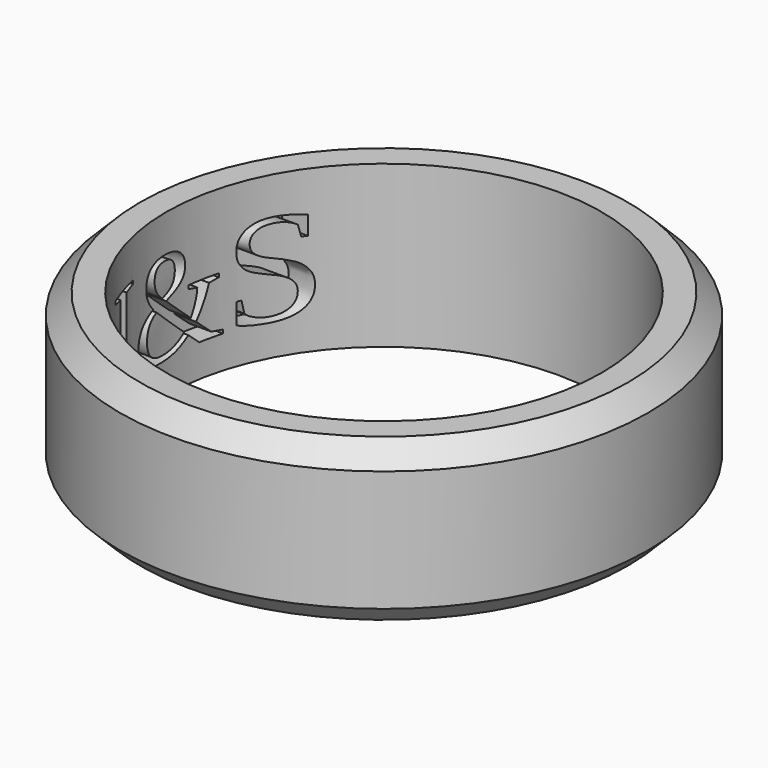
from build123d import *

# Parameters (mm, degrees)
F0_R         = 13
F0_R_2       = 10.8
F1_DEPTH     = 8
F2_TEXT_SIZE = 6.8446094196
F3_DEPTH     = 13.001
F4_R         = 13
F4_R_2       = 11.8668611941
F5_DEPTH     = 25
F6_R         = 13.1
F6_R_2       = 11.8668611941
F7_DEPTH     = 8
F8_SIZE      = 1
F9_SIZE      = 1


# Not quite as in the source:
# - Text() gives the source's letters only with a copy of the font that has no kerning and outlines rounded to 1/6400 em; it was checked with that copy


with BuildPart() as f1:
    # F0 (on Top) → F1 (new body)
    with BuildSketch(Plane.XY):
        Circle(F0_R)
        Circle(F0_R_2, mode=Mode.SUBTRACT)
    extrude(amount=F1_DEPTH)

    # F2 (on Right) → F3 (cut, through all)
    with BuildSketch(Plane.YZ):
        with Locations((-7.1465540677, 1.6091747675)):
            Text('H&S', F2_TEXT_SIZE, font='Tinos', text_align=(TextAlign.LEFT, TextAlign.BOTTOM))
    extrude(amount=-F3_DEPTH, mode=Mode.SUBTRACT)

    # F4 (on face) → F5 (cut)
    with BuildSketch(Plane.XY.offset(8)):
        Circle(F4_R)
        Circle(F4_R_2, mode=Mode.SUBTRACT)
    extrude(amount=-F5_DEPTH, mode=Mode.SUBTRACT)

    # F6 (on face) → F7 (join)
    with BuildSketch(Plane(origin=(0, 0, 0), x_dir=(1, 0, 0), z_dir=(0, 0, -1))):
        Circle(F6_R)
        Circle(F6_R_2, mode=Mode.SUBTRACT)
    extrude(amount=-F7_DEPTH)

    # F8
    f8_edges = [f1.edges().sort_by_distance(p)[0] for p in [
        (-13.1, 0, 0),
    ]]
    chamfer(f8_edges, length=F8_SIZE)

    # F9
    f9_edges = [f1.edges().sort_by_distance(p)[0] for p in [
        (-13.1, 0, 8),
    ]]
    chamfer(f9_edges, length=F9_SIZE)


solid = f1.part
